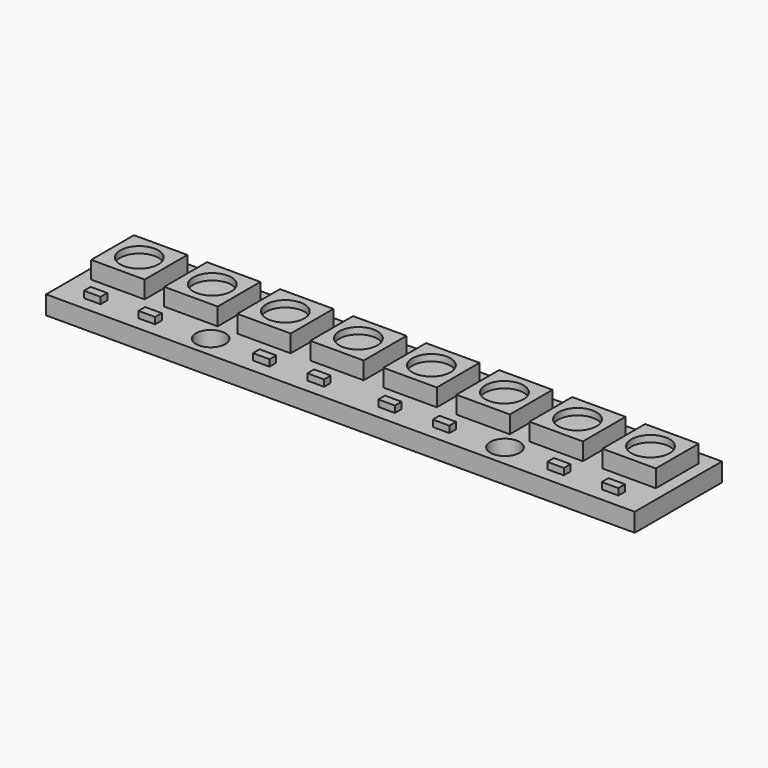
from build123d import *

# Parameters (mm, degrees)
F0_W     = 54
F0_H     = 10
F0_R     = 1.35
F2_DEPTH = 1.7
F1_W     = 4.9
F1_H     = 4.9
F1_R     = 1.75
F3_DEPTH = 1.6
F4_DEPTH = 1
F1_W_2   = 1.524
F1_H_2   = 0.762
F5_DEPTH = 0.6


with BuildPart() as f2:
    # F0 (on Top) → F2 (new body)
    with BuildSketch(Plane.XY):
        with Locations((0, 5)):
            Rectangle(F0_W, F0_H)
        with Locations((-13.5, 2)):
            Circle(F0_R, mode=Mode.SUBTRACT)
        with Locations((13.5, 2)):
            Circle(F0_R, mode=Mode.SUBTRACT)
    extrude(amount=-F2_DEPTH)


with BuildPart() as f3:
    # F1 (on Top) → F3 (new body)
    with BuildSketch(Plane.XY):
        with Locations((-23.45, 6.25)):
            Rectangle(F1_W, F1_H)
        with Locations((-23.45, 6.25)):
            Circle(F1_R, mode=Mode.SUBTRACT)
    extrude(amount=F3_DEPTH)

    # F1 (on Top) → F4, piece 8 (join)
    with BuildSketch(Plane.XY):
        with Locations((-23.45, 6.25)):
            Circle(F1_R)
    extrude(amount=F4_DEPTH)


with BuildPart() as f3b:
    # F1 (on Top) → F3, piece 2 (new body)
    with BuildSketch(Plane.XY):
        with Locations((-16.75, 6.25)):
            Rectangle(F1_W, F1_H)
        with Locations((-16.75, 6.25)):
            Circle(F1_R, mode=Mode.SUBTRACT)
    extrude(amount=F3_DEPTH)

    # F1 (on Top) → F4, piece 7 (join)
    with BuildSketch(Plane.XY):
        with Locations((-16.75, 6.25)):
            Circle(F1_R)
    extrude(amount=F4_DEPTH)


with BuildPart() as f3c:
    # F1 (on Top) → F3, piece 3 (new body)
    with BuildSketch(Plane.XY):
        with Locations((-10.05, 6.25)):
            Rectangle(F1_W, F1_H)
        with Locations((-10.05, 6.25)):
            Circle(F1_R, mode=Mode.SUBTRACT)
    extrude(amount=F3_DEPTH)

    # F1 (on Top) → F4, piece 6 (join)
    with BuildSketch(Plane.XY):
        with Locations((-10.05, 6.25)):
            Circle(F1_R)
    extrude(amount=F4_DEPTH)


with BuildPart() as f3d:
    # F1 (on Top) → F3, piece 4 (new body)
    with BuildSketch(Plane.XY):
        with Locations((-3.35, 6.25)):
            Rectangle(F1_W, F1_H)
        with Locations((-3.35, 6.25)):
            Circle(F1_R, mode=Mode.SUBTRACT)
    extrude(amount=F3_DEPTH)

    # F1 (on Top) → F4, piece 5 (join)
    with BuildSketch(Plane.XY):
        with Locations((-3.35, 6.25)):
            Circle(F1_R)
    extrude(amount=F4_DEPTH)


with BuildPart() as f3e:
    # F1 (on Top) → F3, piece 5 (new body)
    with BuildSketch(Plane.XY):
        with Locations((3.35, 6.25)):
            Rectangle(F1_W, F1_H)
        with Locations((3.35, 6.25)):
            Circle(F1_R, mode=Mode.SUBTRACT)
    extrude(amount=F3_DEPTH)

    # F1 (on Top) → F4, piece 4 (join)
    with BuildSketch(Plane.XY):
        with Locations((3.35, 6.25)):
            Circle(F1_R)
    extrude(amount=F4_DEPTH)


with BuildPart() as f3f:
    # F1 (on Top) → F3, piece 6 (new body)
    with BuildSketch(Plane.XY):
        with Locations((10.05, 6.25)):
            Rectangle(F1_W, F1_H)
        with Locations((10.05, 6.25)):
            Circle(F1_R, mode=Mode.SUBTRACT)
    extrude(amount=F3_DEPTH)

    # F1 (on Top) → F4, piece 3 (join)
    with BuildSketch(Plane.XY):
        with Locations((10.05, 6.25)):
            Circle(F1_R)
    extrude(amount=F4_DEPTH)


with BuildPart() as f3g:
    # F1 (on Top) → F3, piece 7 (new body)
    with BuildSketch(Plane.XY):
        with Locations((16.75, 6.25)):
            Rectangle(F1_W, F1_H)
        with Locations((16.75, 6.25)):
            Circle(F1_R, mode=Mode.SUBTRACT)
    extrude(amount=F3_DEPTH)

    # F1 (on Top) → F4, piece 2 (join)
    with BuildSketch(Plane.XY):
        with Locations((16.75, 6.25)):
            Circle(F1_R)
    extrude(amount=F4_DEPTH)


with BuildPart() as f3h:
    # F1 (on Top) → F3, piece 8 (new body)
    with BuildSketch(Plane.XY):
        with Locations((23.45, 6.25)):
            Rectangle(F1_W, F1_H)
        with Locations((23.45, 6.25)):
            Circle(F1_R, mode=Mode.SUBTRACT)
    extrude(amount=F3_DEPTH)

    # F1 (on Top) → F4 (join)
    with BuildSketch(Plane.XY):
        with Locations((23.45, 6.25)):
            Circle(F1_R)
    extrude(amount=F4_DEPTH)


with BuildPart() as f5:
    # F1 (on Top) → F5 (new body)
    with BuildSketch(Plane.XY):
        with Locations((23.75, 1.619)):
            Rectangle(F1_W_2, F1_H_2)
    extrude(amount=F5_DEPTH)


with BuildPart() as f5b:
    # F1 (on Top) → F5, piece 2 (new body)
    with BuildSketch(Plane.XY):
        with Locations((18.75, 1.619)):
            Rectangle(F1_W_2, F1_H_2)
    extrude(amount=F5_DEPTH)


with BuildPart() as f5c:
    # F1 (on Top) → F5, piece 3 (new body)
    with BuildSketch(Plane.XY):
        with Locations((8.25, 1.619)):
            Rectangle(F1_W_2, F1_H_2)
    extrude(amount=F5_DEPTH)


with BuildPart() as f5d:
    # F1 (on Top) → F5, piece 4 (new body)
    with BuildSketch(Plane.XY):
        with Locations((3.25, 1.619)):
            Rectangle(F1_W_2, F1_H_2)
    extrude(amount=F5_DEPTH)


with BuildPart() as f5e:
    # F1 (on Top) → F5, piece 5 (new body)
    with BuildSketch(Plane.XY):
        with Locations((-3.25, 1.619)):
            Rectangle(F1_W_2, F1_H_2)
    extrude(amount=F5_DEPTH)


with BuildPart() as f5f:
    # F1 (on Top) → F5, piece 6 (new body)
    with BuildSketch(Plane.XY):
        with Locations((-8.25, 1.619)):
            Rectangle(F1_W_2, F1_H_2)
    extrude(amount=F5_DEPTH)


with BuildPart() as f5g:
    # F1 (on Top) → F5, piece 7 (new body)
    with BuildSketch(Plane.XY):
        with Locations((-18.75, 1.619)):
            Rectangle(F1_W_2, F1_H_2)
    extrude(amount=F5_DEPTH)


with BuildPart() as f5h:
    # F1 (on Top) → F5, piece 8 (new body)
    with BuildSketch(Plane.XY):
        with Locations((-23.75, 1.619)):
            Rectangle(F1_W_2, F1_H_2)
    extrude(amount=F5_DEPTH)


solid = Compound([f2.part, f3.part, f3b.part, f3c.part, f3d.part, f3e.part, f3f.part, f3g.part, f3h.part, f5.part, f5b.part, f5c.part, f5d.part, f5e.part, f5f.part, f5g.part, f5h.part])
